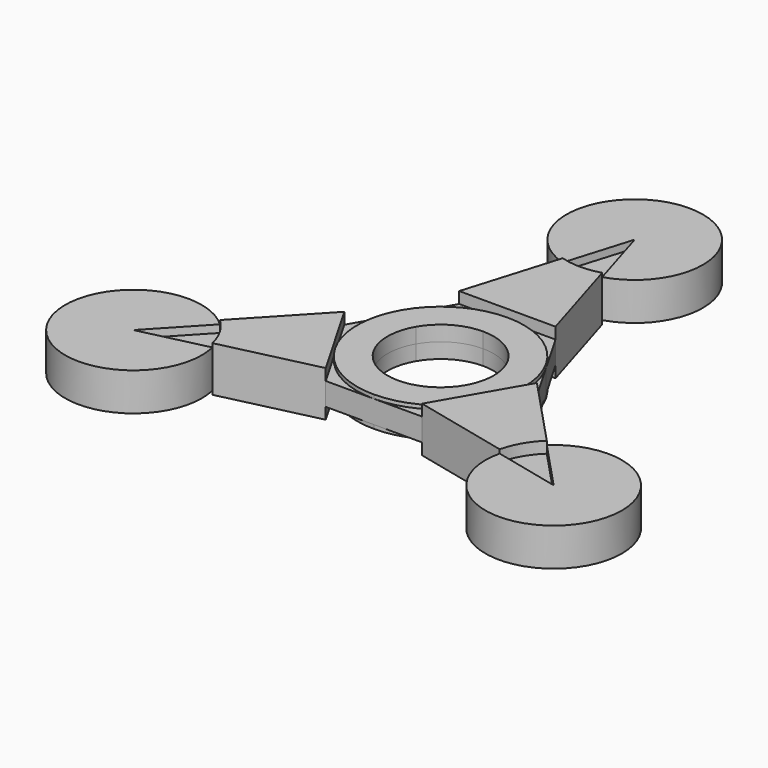
from build123d import *

# Parameters (mm, degrees)
F1_DEPTH      = 3.175
F1_DEPTH_BACK = 3.175
F2_DEPTH      = 2.38125
F2_DEPTH_BACK = 2.38125
F3_DEPTH      = 4.7625
F3_DEPTH_BACK = 4.7625
F4_DEPTH      = 3.96875
F4_DEPTH_BACK = 3.96875
F5_DEPTH      = 2.38125
F5_DEPTH_BACK = 2.38125


# Not quite as in the source:
# - a length typed as a fraction of an inch, garbled in the dataset ("3 / 203.2 mm" for 3/8 in), is restored


with BuildPart() as f1:
    # F0 (on Top) → F1 (new body, two sides)
    with BuildSketch(Plane.XY) as f1_sk:
        with BuildLine():
            Line((0, -17.4625), (0, -11.1125))
            ThreePointArc((0, -11.1125), (-5.55625, -9.6237072996), (-9.6237072996, -5.55625))
            Line((-9.6237072996, -5.55625), (-15.1229686136, -8.73125))
            ThreePointArc((-15.1229686303, -8.731249971), (-8.7312500094, -15.1229686082), (1.18e-08, -17.4625))
        make_face()
        with BuildLine():
            ThreePointArc((-9.6237072996, 5.55625), (-5.55625, 9.6237072996), (0, 11.1125))
            Line((0, 11.1125), (0, 17.4625))
            ThreePointArc((0, 17.4625), (-8.7312499932, 15.1229686175), (-15.1229686057, 8.7312500136))
            Line((-15.1229686136, 8.73125), (-9.6237072996, 5.55625))
        make_face()
        with BuildLine():
            ThreePointArc((-9.6237072996, -5.55625), (-11.1125, 0), (-9.6237072996, 5.55625))
            Line((-9.6237072996, 5.55625), (-15.1229686136, 8.73125))
            ThreePointArc((-15.1229686057, 8.7312500136), (-17.4625, 2.46e-08), (-15.1229686303, -8.731249971))
            Line((-15.1229686136, -8.73125), (-9.6237072996, -5.55625))
        make_face()
        with BuildLine():
            ThreePointArc((0, 11.1125), (5.55625, 9.6237072996), (9.6237072996, 5.55625))
            Line((9.6237072996, 5.55625), (15.1229686136, 8.73125))
            ThreePointArc((15.1229686421, 8.7312499507), (8.7312500247, 15.1229685993), (0, 17.4625))
            Line((0, 17.4625), (0, 11.1125))
        make_face()
        with BuildLine():
            ThreePointArc((9.6237072996, 5.55625), (10.7338507446, 2.8761266387), (11.1125, 0))
            ThreePointArc((11.1125, 0), (10.7338507446, -2.8761266387), (9.6237072996, -5.55625))
            Line((9.6237072996, -5.55625), (15.1229686136, -8.73125))
            ThreePointArc((15.1229686466, -8.7312499429), (16.8674797501, -4.5196275433), (17.4625, 0))
            ThreePointArc((17.4625, 0), (16.8674797489, 4.5196275476), (15.1229686421, 8.7312499507))
            Line((15.1229686136, 8.73125), (9.6237072996, 5.55625))
        make_face()
        with BuildLine():
            Line((15.1229686136, -8.73125), (9.6237072996, -5.55625))
            ThreePointArc((9.6237072996, -5.55625), (5.55625, -9.6237072996), (0, -11.1125))
            Line((0, -11.1125), (0, -17.4625))
            ThreePointArc((1.18e-08, -17.4625), (8.7312500336, -15.1229685942), (15.1229686466, -8.7312499429))
        make_face()
    extrude(amount=-F1_DEPTH)
    extrude(f1_sk.sketch, amount=F1_DEPTH_BACK)

    # F0 (on Top) → F2 (join, two sides)
    with BuildSketch(Plane.XY) as f2_sk:
        with BuildLine():
            ThreePointArc((-15.1229686303, -8.731249971), (-17.4625, 2.46e-08), (-15.1229686057, 8.7312500136))
            Line((-15.1229686057, 8.7312500136), (-20.1639581514, 0))
            Line((-20.1639581514, 0), (-15.1229686303, -8.731249971))
        make_face()
        with BuildLine():
            Line((-10.0819790757, -17.4625), (1.18e-08, -17.4625))
            ThreePointArc((1.18e-08, -17.4625), (-8.7312500094, -15.1229686082), (-15.1229686303, -8.731249971))
            Line((-15.1229686303, -8.731249971), (-10.0819790757, -17.4625))
        make_face()
        with BuildLine():
            ThreePointArc((-15.1229686057, 8.7312500136), (-8.7312499932, 15.1229686175), (0, 17.4625))
            Line((0, 17.4625), (-10.0819790757, 17.4625))
            Line((-10.0819790757, 17.4625), (-15.1229686057, 8.7312500136))
        make_face()
        with BuildLine():
            ThreePointArc((0, 17.4625), (8.7312500247, 15.1229685993), (15.1229686421, 8.7312499507))
            Line((15.1229686421, 8.7312499507), (10.0819790757, 17.4625))
            Line((10.0819790757, 17.4625), (0, 17.4625))
        make_face()
        with BuildLine():
            Line((10.0819790757, -17.4625), (15.1229686466, -8.7312499429))
            ThreePointArc((15.1229686466, -8.7312499429), (8.7312500336, -15.1229685942), (1.18e-08, -17.4625))
            Line((1.18e-08, -17.4625), (10.0819790757, -17.4625))
        make_face()
        with BuildLine():
            Line((20.1639581514, 0), (15.1229686421, 8.7312499507))
            ThreePointArc((15.1229686421, 8.7312499507), (16.8674797489, 4.5196275476), (17.4625, 0))
            ThreePointArc((17.4625, 0), (16.8674797501, -4.5196275433), (15.1229686466, -8.7312499429))
            Line((15.1229686466, -8.7312499429), (20.1639581514, 0))
        make_face()
    extrude(amount=F2_DEPTH)
    extrude(f2_sk.sketch, amount=-F2_DEPTH_BACK)


with BuildPart() as f3:
    # F0 (on Top) → F3 (new body, two sides)
    with BuildSketch(Plane.XY) as f3_sk:
        with BuildLine():
            Line((31.6207525557, -18.25625), (15.1229686136, -8.73125))
            Line((15.1229686466, -8.7312499429), (10.0819790757, -17.4625))
            Line((10.0819790757, -17.4625), (30.0825773544, -22.1438584325))
            ThreePointArc((30.0825773544, -22.1438584325), (30.7086953597, -20.1434867173), (31.6207525557, -18.25625))
        make_face()
        with BuildLine():
            Line((20.1639581514, 0), (15.1229686466, -8.7312499429))
            Line((15.1229686136, -8.73125), (31.6207525557, -18.25625))
            ThreePointArc((31.6207525557, -18.25625), (32.7991188978, -16.52276694), (34.2184326175, -14.9803469839))
            Line((34.2184326175, -14.9803469839), (20.1639581514, 0))
        make_face()
    extrude(amount=F3_DEPTH)
    extrude(f3_sk.sketch, amount=-F3_DEPTH_BACK)


with BuildPart() as f3b:
    # F0 (on Top) → F3, piece 2 (new body, two sides)
    with BuildSketch(Plane.XY) as f3_2_sk:
        with BuildLine():
            Line((0, 36.5125), (0, 17.4625))
            Line((0, 17.4625), (10.0819790757, 17.4625))
            Line((10.0819790757, 17.4625), (4.1358552632, 37.1242054164))
            ThreePointArc((4.1358552632, 37.1242054164), (2.0904235381, 36.6662536572), (0, 36.5125))
        make_face()
        with BuildLine():
            Line((-10.0819790757, 17.4625), (0, 17.4625))
            Line((0, 17.4625), (0, 36.5125))
            ThreePointArc((0, 36.5125), (-2.0904235381, 36.6662536572), (-4.1358552632, 37.1242054164))
            Line((-4.1358552632, 37.1242054164), (-10.0819790757, 17.4625))
        make_face()
    extrude(amount=F3_DEPTH)
    extrude(f3_2_sk.sketch, amount=-F3_DEPTH_BACK)


with BuildPart() as f3c:
    # F0 (on Top) → F3, piece 3 (new body, two sides)
    with BuildSketch(Plane.XY) as f3_3_sk:
        with BuildLine():
            Line((-10.0819790757, -17.4625), (-15.1229686303, -8.731249971))
            Line((-15.1229686136, -8.73125), (-31.6207525557, -18.25625))
            ThreePointArc((-31.6207525557, -18.25625), (-30.7086953597, -20.1434867173), (-30.0825773544, -22.1438584325))
            Line((-30.0825773544, -22.1438584325), (-10.0819790757, -17.4625))
        make_face()
        with BuildLine():
            Line((-31.6207525557, -18.25625), (-15.1229686136, -8.73125))
            Line((-15.1229686303, -8.731249971), (-20.1639581514, 0))
            Line((-20.1639581514, 0), (-34.2184326175, -14.9803469839))
            ThreePointArc((-34.2184326175, -14.9803469839), (-32.7991188978, -16.52276694), (-31.6207525557, -18.25625))
        make_face()
    extrude(amount=F3_DEPTH)
    extrude(f3_3_sk.sketch, amount=-F3_DEPTH_BACK)


with BuildPart() as f4:
    # F0 (on Top) → F4 (new body, two sides)
    with BuildSketch(Plane.XY) as f4_sk:
        with BuildLine():
            Line((0, 50.8), (4.1358552632, 37.1242054164))
            ThreePointArc((4.1358552632, 37.1242054164), (11.4722205419, 42.2840847768), (14.2875, 50.8))
            ThreePointArc((14.2875, 50.8), (-8.5159152232, 62.2722205419), (-4.1358552632, 37.1242054164))
            Line((-4.1358552632, 37.1242054164), (0, 50.8))
        make_face()
    extrude(amount=F4_DEPTH)
    extrude(f4_sk.sketch, amount=-F4_DEPTH_BACK)


with BuildPart() as f4b:
    # F0 (on Top) → F4, piece 2 (new body, two sides)
    with BuildSketch(Plane.XY) as f4_2_sk:
        with BuildLine():
            ThreePointArc((-29.7065905122, -25.4), (-29.8008984736, -23.7611113512), (-30.0825773544, -22.1438584325))
            Line((-30.0825773544, -22.1438584325), (-43.9940905122, -25.4))
            Line((-43.9940905122, -25.4), (-34.2184326175, -14.9803469839))
            ThreePointArc((-34.2184326175, -14.9803469839), (-57.105199703, -31.0772768155), (-29.7065905122, -25.4))
        make_face()
    extrude(amount=F4_DEPTH)
    extrude(f4_2_sk.sketch, amount=-F4_DEPTH_BACK)


with BuildPart() as f4c:
    # F0 (on Top) → F4, piece 3 (new body, two sides)
    with BuildSketch(Plane.XY) as f4_3_sk:
        with BuildLine():
            ThreePointArc((58.2815905122, -25.4), (49.6713673277, -12.2888908093), (34.2184326175, -14.9803469839))
            Line((34.2184326175, -14.9803469839), (43.9940905122, -25.4))
            Line((43.9940905122, -25.4), (30.0825773544, -22.1438584325))
            ThreePointArc((30.0825773544, -22.1438584325), (42.3552018634, -39.5931920387), (58.2815905122, -25.4))
        make_face()
    extrude(amount=F4_DEPTH)
    extrude(f4_3_sk.sketch, amount=-F4_DEPTH_BACK)


with BuildPart() as f5:
    # F0 (on Top) → F5 (new body, two sides)
    with BuildSketch(Plane.XY) as f5_sk:
        with BuildLine():
            Line((43.9940905122, -25.4), (31.6207525557, -18.25625))
            ThreePointArc((31.6207525557, -18.25625), (30.7086953597, -20.1434867173), (30.0825773544, -22.1438584325))
            Line((30.0825773544, -22.1438584325), (43.9940905122, -25.4))
        make_face()
        with BuildLine():
            ThreePointArc((34.2184326175, -14.9803469839), (32.7991188978, -16.52276694), (31.6207525557, -18.25625))
            Line((31.6207525557, -18.25625), (43.9940905122, -25.4))
            Line((43.9940905122, -25.4), (34.2184326175, -14.9803469839))
        make_face()
    extrude(amount=F5_DEPTH)
    extrude(f5_sk.sketch, amount=-F5_DEPTH_BACK)


with BuildPart() as f5b:
    # F0 (on Top) → F5, piece 2 (new body, two sides)
    with BuildSketch(Plane.XY) as f5_2_sk:
        with BuildLine():
            Line((0, 50.8), (0, 36.5125))
            ThreePointArc((0, 36.5125), (2.0904235381, 36.6662536572), (4.1358552632, 37.1242054164))
            Line((4.1358552632, 37.1242054164), (0, 50.8))
        make_face()
        with BuildLine():
            ThreePointArc((-4.1358552632, 37.1242054164), (-2.0904235381, 36.6662536572), (0, 36.5125))
            Line((0, 36.5125), (0, 50.8))
            Line((0, 50.8), (-4.1358552632, 37.1242054164))
        make_face()
    extrude(amount=F5_DEPTH)
    extrude(f5_2_sk.sketch, amount=-F5_DEPTH_BACK)


with BuildPart() as f5c:
    # F0 (on Top) → F5, piece 3 (new body, two sides)
    with BuildSketch(Plane.XY) as f5_3_sk:
        with BuildLine():
            Line((-43.9940905122, -25.4), (-31.6207525557, -18.25625))
            ThreePointArc((-31.6207525557, -18.25625), (-32.7991188978, -16.52276694), (-34.2184326175, -14.9803469839))
            Line((-34.2184326175, -14.9803469839), (-43.9940905122, -25.4))
        make_face()
        with BuildLine():
            ThreePointArc((-30.0825773544, -22.1438584325), (-30.7086953597, -20.1434867173), (-31.6207525557, -18.25625))
            Line((-31.6207525557, -18.25625), (-43.9940905122, -25.4))
            Line((-43.9940905122, -25.4), (-30.0825773544, -22.1438584325))
        make_face()
    extrude(amount=F5_DEPTH)
    extrude(f5_3_sk.sketch, amount=-F5_DEPTH_BACK)


solid = Compound([f1.part, f3.part, f3b.part, f3c.part, f4.part, f4b.part, f4c.part, f5.part, f5b.part, f5c.part])
